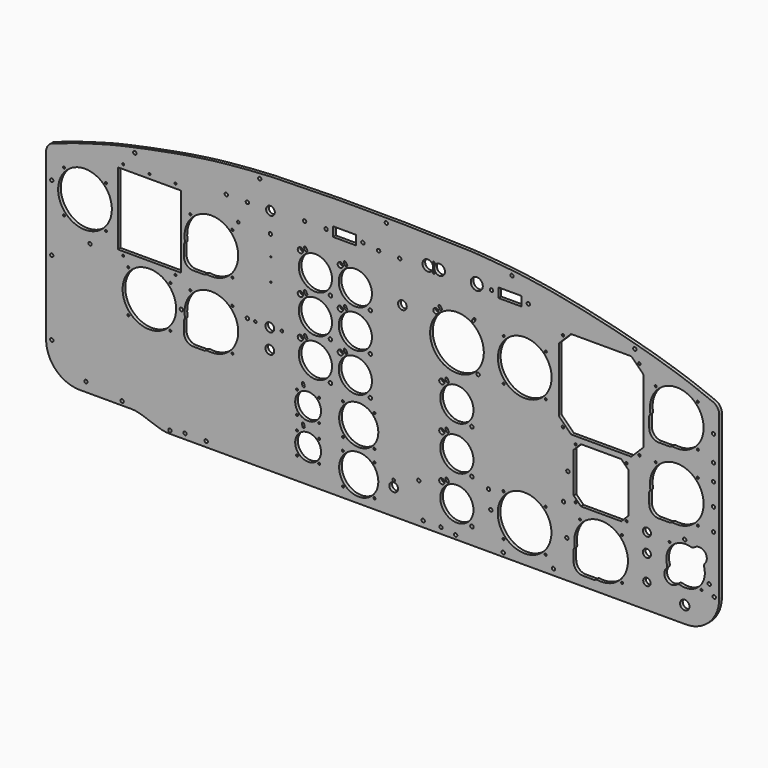
from build123d import *

# Parameters (mm, degrees)
F0_R     = 2.5
F0_R_2   = 1.5
F0_R_3   = 29.25
F0_R_4   = 19.3
F0_R_5   = 39.95
F0_R_6   = 2.6
F0_R_7   = 6.5
F0_R_8   = 2
F0_R_9   = 24.8
F0_R_10  = 3.95
F0_R_11  = 40.1
F0_R_12  = 5.5
F0_R_13  = 7
F0_R_14  = 6
F0_W     = 94
F0_H     = 108
F0_R_15  = 1
F0_W_2   = 34
F0_H_2   = 14
F0_R_16  = 1.8
F0_R_17  = 8
F0_R_18  = 9
F1_DEPTH = 5


# Not quite as in the source:
# - ends of sketch curves that miss each other by under 0.0002 mm in the source are joined
# - a feature names something its author has since deleted; it is built from what else it names


with BuildPart() as f1:
    # F0 (on Front) → F1 (new body)
    with BuildSketch(Plane.XZ):
        with BuildLine():
            ThreePointArc((135.741569039, 191.2079776505), (132.6141103531, 191.3792452145), (129.4850340278, 191.5178517119))
            ThreePointArc((129.4850340278, 191.5178517119), (-17.7264600255, 194.6267238973), (-164.9547639998, 192.4551859949))
            Line((-164.9547639998, 192.4551859949), (-191.066396, 190.888488))
            ThreePointArc((-191.066396, 190.888488), (-199.9950090203, 190.2859144937), (-208.9136419356, 189.5502432845))
            Line((-208.9136419356, 189.5502432845), (-232.326729, 187.443066))
            ThreePointArc((-232.326729, 187.443066), (-249.9687704393, 185.5919994012), (-267.5483811225, 183.2202148163))
            Line((-267.5483811225, 183.2202148163), (-288.605712, 180.061615))
            ThreePointArc((-288.605712, 180.061615), (-299.9814935886, 178.2434149523), (-311.3202700448, 176.2071422363))
            Line((-311.3202700448, 176.2071422363), (-344.055131, 170.003487))
            ThreePointArc((-344.055131, 170.003487), (-349.9940173558, 168.8469464334), (-355.9209391639, 167.6305767785))
            Line((-355.9209391639, 167.6305767785), (-380.749966, 162.404369))
            ThreePointArc((-380.749966, 162.404369), (-399.923291883, 158.0393315675), (-418.9432839055, 153.0483516623))
            Line((-418.9432839055, 153.0483516623), (-436.763326, 148.05874))
            ThreePointArc((-436.763326, 148.05874), (-449.9540896327, 144.201879695), (-463.0530571075, 140.0439153256))
            Line((-463.0530571075, 140.0439153256), (-492.340506, 130.376708))
            ThreePointArc((-492.340506, 130.376708), (-499.6985161403, 124.9082347034), (-502.5, 116.179191))
            Line((-502.5, 116.179191), (-502.5, -130.647528))
            ThreePointArc((-502.5, -130.647528), (-487.8553390593, -166.0028670593), (-452.5, -180.647528))
            Line((-452.5, -180.647528), (-375.801279, -180.647528))
            ThreePointArc((-375.801279, -180.647528), (-367.6120980534, -181.3227136017), (-359.6440857893, -183.3300353831))
            Line((-359.6440857893, -183.3300353831), (-334.355914, -191.965021))
            ThreePointArc((-334.355914, -191.965021), (-326.3879017872, -193.9723424247), (-318.198721, -194.647528))
            Line((-318.198721, -194.647528), (452.5, -194.647528))
            ThreePointArc((452.5, -194.647528), (487.8553390593, -180.0028670593), (502.5, -144.647528))
            Line((502.5, -144.647528), (502.5, 97.162105))
            ThreePointArc((502.5, 97.162105), (499.8924727989, 105.6135319758), (492.976450943, 111.1266488547))
            Line((492.976450943, 111.1266488547), (469.730257, 120.173737))
            ThreePointArc((469.730257, 120.173737), (449.8769209382, 127.4999158755), (429.7775799751, 134.1214219196))
            Line((429.7775799751, 134.1214219196), (410.573025, 140.074834))
            ThreePointArc((410.573025, 140.074834), (399.9715720426, 143.2544076566), (389.3132729084, 146.2378876609))
            Line((389.3132729084, 146.2378876609), (360.903911, 153.908416))
            ThreePointArc((360.903911, 153.908416), (349.9742295543, 156.7493500292), (338.9930159808, 159.3840779165))
            Line((338.9930159808, 159.3840779165), (308.383551, 166.424255))
            ThreePointArc((308.383551, 166.424255), (299.9870413401, 168.2921835026), (291.5646160829, 170.0395484146))
            Line((291.5646160829, 170.0395484146), (264.271898, 175.498092))
            ThreePointArc((264.271898, 175.498092), (249.9695922042, 178.1786072411), (235.6064889537, 180.5114976916))
            Line((235.6064889537, 180.5114976916), (217.548382, 183.220214))
            ThreePointArc((217.548382, 183.220214), (199.9687714246, 185.5919992831), (182.3267300249, 187.4430662765))
            Line((182.3267300249, 187.4430662765), (158.913642, 189.550244))
            ThreePointArc((158.913642, 189.550244), (149.9950095181, 190.2859144564), (141.0663969549, 190.8884872484))
            Line((141.0663969549, 190.8884872484), (135.741569039, 191.2079776505))
        make_face()
        with Locations((-389, -174.647528)):
            Circle(F0_R, mode=Mode.SUBTRACT)
        with Locations((-443, -166.647528)):
            Circle(F0_R, mode=Mode.SUBTRACT)
        with Locations((-317.5, -190.147528)):
            Circle(F0_R, mode=Mode.SUBTRACT)
        with Locations((-295, -186.647528)):
            Circle(F0_R, mode=Mode.SUBTRACT)
        with Locations((-263.5, -186.647528)):
            Circle(F0_R, mode=Mode.SUBTRACT)
        with Locations((-494, -128.647528)):
            Circle(F0_R, mode=Mode.SUBTRACT)
        with Locations((-127.881654, -161.579183)):
            Circle(F0_R_2, mode=Mode.SUBTRACT)
        with Locations((-59.3, -179.947528)):
            Circle(F0_R_2, mode=Mode.SUBTRACT)
        with Locations((-12.2, -179.947528)):
            Circle(F0_R_2, mode=Mode.SUBTRACT)
        with Locations((-94.718346, -161.579183)):
            Circle(F0_R_2, mode=Mode.SUBTRACT)
        with Locations((-35.75, -156.397528)):
            Circle(F0_R_3, mode=Mode.SUBTRACT)
        with Locations((-127.881654, -128.415874)):
            Circle(F0_R_2, mode=Mode.SUBTRACT)
        with Locations((-127.881654, -107.979183)):
            Circle(F0_R_2, mode=Mode.SUBTRACT)
        with Locations((-111.3, -144.997528)):
            Circle(F0_R_4, mode=Mode.SUBTRACT)
        with Locations((-94.718346, -128.415874)):
            Circle(F0_R_2, mode=Mode.SUBTRACT)
        with Locations((-59.3, -132.847528)):
            Circle(F0_R_2, mode=Mode.SUBTRACT)
        with Locations((-12.2, -132.847528)):
            Circle(F0_R_2, mode=Mode.SUBTRACT)
        with BuildLine():
            ThreePointArc((-116.3510682855, -119.9195418044), (-117.5768700198, -122.0695354275), (-119.7268511404, -120.8437117647))
            Line((-119.7268511404, -120.8437117647), (-120.650987, -117.467919))
            ThreePointArc((-120.650987, -117.467919), (-119.4175845384, -115.3159006328), (-117.2711185731, -116.5589411514))
            Line((-117.2711185731, -116.5589411514), (-116.3510682855, -119.9195418044))
        make_face(mode=Mode.SUBTRACT)
        with Locations((-94.718346, -107.979183)):
            Circle(F0_R_2, mode=Mode.SUBTRACT)
        with Locations((-59.3, -114.947528)):
            Circle(F0_R_2, mode=Mode.SUBTRACT)
        with Locations((-12.2, -114.947528)):
            Circle(F0_R_2, mode=Mode.SUBTRACT)
        with Locations((-379.730896, -58.878425)):
            Circle(F0_R_2, mode=Mode.SUBTRACT)
        with Locations((-316.869103, -58.878425)):
            Circle(F0_R_2, mode=Mode.SUBTRACT)
        with Locations((-494, -17.147528)):
            Circle(F0_R, mode=Mode.SUBTRACT)
        with Locations((-348.3, -27.447528)):
            Circle(F0_R_5, mode=Mode.SUBTRACT)
        with Locations((-300.5, -25.647528)):
            Circle(F0_R, mode=Mode.SUBTRACT)
        with BuildLine():
            ThreePointArc((-264.6933823946, -68.0597605441), (-265.3038534949, -68.4216231267), (-266.002257, -68.547528))
            Line((-266.002257, -68.547528), (-282.6, -68.547528))
            ThreePointArc((-282.6, -68.547528), (-292.6409162928, -64.3884442928), (-296.8, -54.347528))
            Line((-296.8, -54.347528), (-296.8, -38.547528))
            ThreePointArc((-296.8, -38.547528), (-296.6647556198, -37.8245574071), (-296.2773135218, -37.1993645239))
            ThreePointArc((-296.2773135218, -37.1993645239), (-295.3984169479, -35.6450094204), (-295.2834646323, -33.8630821025))
            ThreePointArc((-295.2834646323, -33.8630821025), (-227.5670304906, 1.1277414928), (-261.4973429879, -67.1262479174))
            ThreePointArc((-261.4973429879, -67.1262479174), (-263.1971096036, -67.2446562762), (-264.6933823946, -68.0597605441))
        make_face(mode=Mode.SUBTRACT)
        with Locations((-127.881654, -74.815874)):
            Circle(F0_R_2, mode=Mode.SUBTRACT)
        with Locations((-224.269103, -58.878425)):
            Circle(F0_R_2, mode=Mode.SUBTRACT)
        with Locations((-111.3, -91.397528)):
            Circle(F0_R_4, mode=Mode.SUBTRACT)
        with Locations((-94.718346, -74.815874)):
            Circle(F0_R_2, mode=Mode.SUBTRACT)
        with Locations((-35.75, -91.397528)):
            Circle(F0_R_3, mode=Mode.SUBTRACT)
        with BuildLine():
            ThreePointArc((-116.3510682855, -66.3195418044), (-117.5768700198, -68.4695354275), (-119.7268511404, -67.2437117647))
            Line((-119.7268511404, -67.2437117647), (-120.650987, -63.867919))
            ThreePointArc((-120.650987, -63.867919), (-119.4175845384, -61.7159006328), (-117.2711185731, -62.9589411514))
            Line((-117.2711185731, -62.9589411514), (-116.3510682855, -66.3195418044))
        make_face(mode=Mode.SUBTRACT)
        with Locations((-77.949362, -49.898169)):
            Circle(F0_R_6, mode=Mode.SUBTRACT)
        with Locations((-59.3, -67.847528)):
            Circle(F0_R_2, mode=Mode.SUBTRACT)
        with Locations((-12.2, -67.847528)):
            Circle(F0_R_2, mode=Mode.SUBTRACT)
        with Locations((-18.349362, -49.898169)):
            Circle(F0_R_6, mode=Mode.SUBTRACT)
        with Locations((-168.5, -35.647528)):
            Circle(F0_R_7, mode=Mode.SUBTRACT)
        with Locations((-202, -5.147528)):
            Circle(F0_R, mode=Mode.SUBTRACT)
        with Locations((-190, -5.647528)):
            Circle(F0_R_8, mode=Mode.SUBTRACT)
        with Locations((-168.5, -6.147528)):
            Circle(F0_R_7, mode=Mode.SUBTRACT)
        with Locations((-150.5, -5.147528)):
            Circle(F0_R_8, mode=Mode.SUBTRACT)
        with Locations((-100.400003, -27.447528)):
            Circle(F0_R_9, mode=Mode.SUBTRACT)
        with Locations((-40.800003, -27.447528)):
            Circle(F0_R_9, mode=Mode.SUBTRACT)
        with Locations((-122.850643, -4.996888)):
            Circle(F0_R_10, mode=Mode.SUBTRACT)
        with BuildLine():
            ThreePointArc((-112.6555519379, -1.6024819658), (-113.3428170619, -3.9800283878), (-115.7203567133, -3.2927398419))
            Line((-115.7203567133, -3.2927398419), (-117.410584, -0.227918))
            ThreePointArc((-117.410584, -0.227918), (-116.7164059044, 2.1533814048), (-114.3382438007, 1.4485311076))
            Line((-114.3382438007, 1.4485311076), (-112.6555519379, -1.6024819658))
        make_face(mode=Mode.SUBTRACT)
        with Locations((-63.250643, -4.996888)):
            Circle(F0_R_10, mode=Mode.SUBTRACT)
        with BuildLine():
            ThreePointArc((-53.0555519379, -1.6024819658), (-53.7428170619, -3.9800283878), (-56.1203567133, -3.2927398419))
            Line((-56.1203567133, -3.2927398419), (-57.810584, -0.227918))
            ThreePointArc((-57.810584, -0.227918), (-57.1164059044, 2.1533814048), (-54.7382438007, 1.4485311076))
            Line((-54.7382438007, 1.4485311076), (-53.0555519379, -1.6024819658))
        make_face(mode=Mode.SUBTRACT)
        with Locations((60.5, -185.647528)):
            Circle(F0_R, mode=Mode.SUBTRACT)
        with Locations((87, -185.647528)):
            Circle(F0_R, mode=Mode.SUBTRACT)
        with Locations((109, -188.647528)):
            Circle(F0_R, mode=Mode.SUBTRACT)
        with Locations((16.5, -156.147528)):
            Circle(F0_R_7, mode=Mode.SUBTRACT)
        with Locations((16.5, -146.647528)):
            Circle(F0_R_8, mode=Mode.SUBTRACT)
        with Locations((110.8, -147.347528)):
            Circle(F0_R_9, mode=Mode.SUBTRACT)
        with Locations((180, -188.647528)):
            Circle(F0_R, mode=Mode.SUBTRACT)
        with Locations((180.419104, -170.978425)):
            Circle(F0_R_2, mode=Mode.SUBTRACT)
        with Locations((243.280897, -170.978425)):
            Circle(F0_R_2, mode=Mode.SUBTRACT)
        with Locations((133.250641, -169.798169)):
            Circle(F0_R_6, mode=Mode.SUBTRACT)
        with Locations((54, -135.147528)):
            Circle(F0_R, mode=Mode.SUBTRACT)
        with Locations((88.34936, -124.896888)):
            Circle(F0_R_10, mode=Mode.SUBTRACT)
        with BuildLine():
            ThreePointArc((98.5444510621, -121.5024819658), (97.8571859381, -123.8800283878), (95.4796462867, -123.1927398419))
            Line((95.4796462867, -123.1927398419), (93.789419, -120.127918))
            ThreePointArc((93.789419, -120.127918), (94.4835970956, -117.7466185952), (96.8617591993, -118.4514688924))
            Line((96.8617591993, -118.4514688924), (98.5444510621, -121.5024819658))
        make_face(mode=Mode.SUBTRACT)
        with Locations((161.5, -138.647528)):
            Circle(F0_R, mode=Mode.SUBTRACT)
        with Locations((211.85, -139.547528)):
            Circle(F0_R_11, mode=Mode.SUBTRACT)
        with Locations((158, -112.647528)):
            Circle(F0_R, mode=Mode.SUBTRACT)
        with Locations((133.250641, -104.198169)):
            Circle(F0_R_6, mode=Mode.SUBTRACT)
        with Locations((180.419104, -108.116632)):
            Circle(F0_R_2, mode=Mode.SUBTRACT)
        with Locations((243.280897, -108.116632)):
            Circle(F0_R_2, mode=Mode.SUBTRACT)
        with Locations((255, -185.647528)):
            Circle(F0_R, mode=Mode.SUBTRACT)
        with Locations((357.530897, -170.978425)):
            Circle(F0_R_2, mode=Mode.SUBTRACT)
        with Locations((394.5, -157.647528)):
            Circle(F0_R_12, mode=Mode.SUBTRACT)
        with Locations((451, -169.647528)):
            Circle(F0_R_13, mode=Mode.SUBTRACT)
        with Locations((275, -138.647528)):
            Circle(F0_R, mode=Mode.SUBTRACT)
        with BuildLine():
            ThreePointArc((317.1066176054, -180.1597605441), (316.4961465051, -180.5216231267), (315.797743, -180.647528))
            Line((315.797743, -180.647528), (299.2, -180.647528))
            ThreePointArc((299.2, -180.647528), (289.1590837072, -176.4884442928), (285, -166.447528))
            Line((285, -166.447528), (285, -150.647528))
            ThreePointArc((285, -150.647528), (285.1352443802, -149.9245574071), (285.5226864782, -149.2993645239))
            ThreePointArc((285.5226864782, -149.2993645239), (286.4015830521, -147.7450094204), (286.5165353677, -145.9630821025))
            ThreePointArc((286.5165353677, -145.9630821025), (354.2329695094, -110.9722585072), (320.3026570121, -179.2262479174))
            ThreePointArc((320.3026570121, -179.2262479174), (318.6028903964, -179.3446562762), (317.1066176054, -180.1597605441))
        make_face(mode=Mode.SUBTRACT)
        with Locations((294.669104, -108.116632)):
            Circle(F0_R_2, mode=Mode.SUBTRACT)
        with Locations((357.530897, -108.116632)):
            Circle(F0_R_2, mode=Mode.SUBTRACT)
        with Locations((476, -141.647528)):
            Circle(F0_R_2, mode=Mode.SUBTRACT)
        with Locations((495, -144.647528)):
            Circle(F0_R, mode=Mode.SUBTRACT)
        with Locations((487.5, -130.147528)):
            Circle(F0_R, mode=Mode.SUBTRACT)
        with Locations((394.5, -120.147528)):
            Circle(F0_R_14, mode=Mode.SUBTRACT)
        with BuildLine():
            ThreePointArc((479.9020604453, -110.0282171579), (472.4459566685, -138.3593420507), (444.0197490276, -145.4443149076))
            ThreePointArc((444.0197490276, -145.4443149076), (441.5053900455, -145.3537612476), (439.2652582695, -146.499191303))
            ThreePointArc((439.2652582695, -146.499191303), (423.7813893308, -145.9962507879), (423.4809780694, -130.5071290634))
            ThreePointArc((423.4809780694, -130.5071290634), (424.6556053692, -128.2821680605), (424.5979402014, -125.7668399427))
            ThreePointArc((424.5979402014, -125.7668399427), (432.0540429937, -97.4357142827), (460.4802512467, -90.3507411744))
            ThreePointArc((460.4802512467, -90.3507411744), (462.9946104868, -90.4412958561), (465.2347427305, -89.295865697))
            ThreePointArc((465.2347427305, -89.295865697), (480.7186109317, -89.798806478), (481.0190219306, -105.2879279366))
            ThreePointArc((481.0190219306, -105.2879279366), (479.8443955535, -107.5128892677), (479.9020604453, -110.0282171579))
        make_face(mode=Mode.SUBTRACT)
        with Locations((110.8, -81.747528)):
            Circle(F0_R_9, mode=Mode.SUBTRACT)
        with Locations((88.34936, -59.296888)):
            Circle(F0_R_10, mode=Mode.SUBTRACT)
        with BuildLine():
            ThreePointArc((98.5444510621, -55.9024819658), (97.8571859381, -58.2800283878), (95.4796462867, -57.5927398419))
            Line((95.4796462867, -57.5927398419), (93.789419, -54.527918))
            ThreePointArc((93.789419, -54.527918), (94.4835970956, -52.1466185952), (96.8617591993, -52.8514688924))
            Line((96.8617591993, -52.8514688924), (98.5444510621, -55.9024819658))
        make_face(mode=Mode.SUBTRACT)
        with Locations((110.8, -16.147528)):
            Circle(F0_R_9, mode=Mode.SUBTRACT)
        with Locations((133.250641, -38.598169)):
            Circle(F0_R_6, mode=Mode.SUBTRACT)
        with Locations((270, -92.647528)):
            Circle(F0_R, mode=Mode.SUBTRACT)
        with Locations((287.995773, -87.63635)):
            Circle(F0_R_2, mode=Mode.SUBTRACT)
        with Locations((364.198177, -87.63635)):
            Circle(F0_R_2, mode=Mode.SUBTRACT)
        with Locations((276.5, -50.647528)):
            Circle(F0_R, mode=Mode.SUBTRACT)
        Polygon((285.199997, -19.462587), (295.999987, -8.648008), (356.186954, -8.648008), (367.000807, -19.447999), (366.999997, -79.63586), (356.200003, -90.447049), (295.999997, -90.448008), (285.199997, -79.648008), align=None, mode=Mode.SUBTRACT)
        with Locations((394.5, -92.147528)):
            Circle(F0_R_14, mode=Mode.SUBTRACT)
        with Locations((428.5, -94.147528)):
            Circle(F0_R_2, mode=Mode.SUBTRACT)
        with Locations((451, -83.647528)):
            Circle(F0_R, mode=Mode.SUBTRACT)
        with Locations((470.530897, -58.878425)):
            Circle(F0_R_2, mode=Mode.SUBTRACT)
        with Locations((494, -59.647528)):
            Circle(F0_R, mode=Mode.SUBTRACT)
        with Locations((287.995773, -11.43635)):
            Circle(F0_R_2, mode=Mode.SUBTRACT)
        with Locations((364.195773, -11.43635)):
            Circle(F0_R_2, mode=Mode.SUBTRACT)
        with BuildLine():
            ThreePointArc((430.1066176054, -68.0597605441), (429.4961465051, -68.4216231267), (428.797743, -68.547528))
            Line((428.797743, -68.547528), (412.2, -68.547528))
            ThreePointArc((412.2, -68.547528), (402.1590837072, -64.3884442928), (398, -54.347528))
            Line((398, -54.347528), (398, -38.547528))
            ThreePointArc((398, -38.547528), (398.1352443802, -37.8245574071), (398.5226864782, -37.1993645239))
            ThreePointArc((398.5226864782, -37.1993645239), (399.4015830521, -35.6450094204), (399.5165353677, -33.8630821025))
            ThreePointArc((399.5165353677, -33.8630821025), (467.2329695094, 1.1277414928), (433.3026570121, -67.1262479174))
            ThreePointArc((433.3026570121, -67.1262479174), (431.6028903964, -67.2446562762), (430.1066176054, -68.0597605441))
        make_face(mode=Mode.SUBTRACT)
        with Locations((494, -26.647528)):
            Circle(F0_R, mode=Mode.SUBTRACT)
        with Locations((-379.730896, 3.983368)):
            Circle(F0_R_2, mode=Mode.SUBTRACT)
        with Locations((-437, 16.352472)):
            Circle(F0_R, mode=Mode.SUBTRACT)
        with Locations((-387.3, 17.002472)):
            Circle(F0_R_2, mode=Mode.SUBTRACT)
        with Locations((-475.830896, 41.021575)):
            Circle(F0_R_2, mode=Mode.SUBTRACT)
        with Locations((-412.969103, 41.021575)):
            Circle(F0_R_2, mode=Mode.SUBTRACT)
        with Locations((-316.869103, 3.983368)):
            Circle(F0_R_2, mode=Mode.SUBTRACT)
        with Locations((-287.130896, 3.983368)):
            Circle(F0_R_2, mode=Mode.SUBTRACT)
        with Locations((-309.3, 17.002472)):
            Circle(F0_R_2, mode=Mode.SUBTRACT)
        with Locations((-444.4, 72.452472)):
            Circle(F0_R_11, mode=Mode.SUBTRACT)
        with Locations((-494, 81.352472)):
            Circle(F0_R, mode=Mode.SUBTRACT)
        with BuildLine():
            ThreePointArc((-264.6933823946, 31.8402394559), (-265.3038534949, 31.4783768733), (-266.002257, 31.352472))
            Line((-266.002257, 31.352472), (-282.6, 31.352472))
            ThreePointArc((-282.6, 31.352472), (-292.6409162928, 35.5115557072), (-296.8, 45.552472))
            Line((-296.8, 45.552472), (-296.8, 61.352472))
            ThreePointArc((-296.8, 61.352472), (-296.6647556198, 62.0754425929), (-296.2773135218, 62.7006354761))
            ThreePointArc((-296.2773135218, 62.7006354761), (-295.3984169479, 64.2549905796), (-295.2834646323, 66.0369178975))
            ThreePointArc((-295.2834646323, 66.0369178975), (-227.5670304906, 101.0277414928), (-261.4973429879, 32.7737520826))
            ThreePointArc((-261.4973429879, 32.7737520826), (-263.1971096036, 32.6553437238), (-264.6933823946, 31.8402394559))
        make_face(mode=Mode.SUBTRACT)
        with Locations((-348.3, 76.502472)):
            Rectangle(F0_W, F0_H, mode=Mode.SUBTRACT)
        with Locations((-224.269103, 3.983368)):
            Circle(F0_R_2, mode=Mode.SUBTRACT)
        with Locations((-224.269103, 41.021575)):
            Circle(F0_R_2, mode=Mode.SUBTRACT)
        with Locations((-77.949359, 7.601831)):
            Circle(F0_R_6, mode=Mode.SUBTRACT)
        with Locations((-18.349359, 7.601831)):
            Circle(F0_R_6, mode=Mode.SUBTRACT)
        with Locations((-100.4, 30.052472)):
            Circle(F0_R_9, mode=Mode.SUBTRACT)
        with Locations((-40.8, 30.052472)):
            Circle(F0_R_9, mode=Mode.SUBTRACT)
        with Locations((-167, 53.852472)):
            Circle(F0_R_15, mode=Mode.SUBTRACT)
        with Locations((-167, 86.852472)):
            Circle(F0_R_15, mode=Mode.SUBTRACT)
        with Locations((-122.85064, 52.503112)):
            Circle(F0_R_10, mode=Mode.SUBTRACT)
        with BuildLine():
            ThreePointArc((-112.6555489379, 55.8975180342), (-113.3428140619, 53.5199716122), (-115.7203537133, 54.2072601581))
            Line((-115.7203537133, 54.2072601581), (-117.410581, 57.272082))
            ThreePointArc((-117.410581, 57.272082), (-116.7164029044, 59.6533814048), (-114.3382408007, 58.9485311076))
            Line((-114.3382408007, 58.9485311076), (-112.6555489379, 55.8975180342))
        make_face(mode=Mode.SUBTRACT)
        with Locations((-63.25064, 52.503112)):
            Circle(F0_R_10, mode=Mode.SUBTRACT)
        with Locations((-77.949359, 65.101831)):
            Circle(F0_R_6, mode=Mode.SUBTRACT)
        with BuildLine():
            ThreePointArc((-53.0555489379, 55.8975180342), (-53.7428140619, 53.5199716122), (-56.1203537133, 54.2072601581))
            Line((-56.1203537133, 54.2072601581), (-57.810581, 57.272082))
            ThreePointArc((-57.810581, 57.272082), (-57.1164029044, 59.6533814048), (-54.7382408007, 58.9485311076))
            Line((-54.7382408007, 58.9485311076), (-53.0555489379, 55.8975180342))
        make_face(mode=Mode.SUBTRACT)
        with Locations((-18.349359, 65.101831)):
            Circle(F0_R_6, mode=Mode.SUBTRACT)
        with Locations((-100.4, 87.552472)):
            Circle(F0_R_9, mode=Mode.SUBTRACT)
        with Locations((-40.8, 87.552472)):
            Circle(F0_R_9, mode=Mode.SUBTRACT)
        with Locations((-475.830896, 103.883368)):
            Circle(F0_R_2, mode=Mode.SUBTRACT)
        with Locations((-412.969103, 103.883368)):
            Circle(F0_R_2, mode=Mode.SUBTRACT)
        with Locations((-387.3, 137.002472)):
            Circle(F0_R_2, mode=Mode.SUBTRACT)
        with Locations((-287.130896, 103.883368)):
            Circle(F0_R_2, mode=Mode.SUBTRACT)
        with Locations((-348.3, 137.002472)):
            Circle(F0_R_2, mode=Mode.SUBTRACT)
        with Locations((-309.3, 137.002472)):
            Circle(F0_R_2, mode=Mode.SUBTRACT)
        with Locations((-370, 157.667106)):
            Circle(F0_R, mode=Mode.SUBTRACT)
        with Locations((-224.269103, 103.883368)):
            Circle(F0_R_2, mode=Mode.SUBTRACT)
        with Locations((-215.5, 116.852472)):
            Circle(F0_R_8, mode=Mode.SUBTRACT)
        with Locations((-167.5, 116.852472)):
            Circle(F0_R, mode=Mode.SUBTRACT)
        with Locations((-122.85064, 110.003112)):
            Circle(F0_R_10, mode=Mode.SUBTRACT)
        with BuildLine():
            ThreePointArc((-112.6555489379, 113.3975180342), (-113.3428140619, 111.0199716122), (-115.7203537133, 111.7072601581))
            Line((-115.7203537133, 111.7072601581), (-117.410581, 114.772082))
            ThreePointArc((-117.410581, 114.772082), (-116.7164029044, 117.1533814048), (-114.3382408007, 116.4485311076))
            Line((-114.3382408007, 116.4485311076), (-112.6555489379, 113.3975180342))
        make_face(mode=Mode.SUBTRACT)
        with Locations((-63.25064, 110.003112)):
            Circle(F0_R_10, mode=Mode.SUBTRACT)
        with BuildLine():
            ThreePointArc((-53.0555489379, 113.3975180342), (-53.7428140619, 111.0199716122), (-56.1203537133, 111.7072601581))
            Line((-56.1203537133, 111.7072601581), (-57.810581, 114.772082))
            ThreePointArc((-57.810581, 114.772082), (-57.1164029044, 117.1533814048), (-54.7382408007, 116.4485311076))
            Line((-54.7382408007, 116.4485311076), (-53.0555489379, 113.3975180342))
        make_face(mode=Mode.SUBTRACT)
        with Locations((-233.5, 147.352472)):
            Circle(F0_R, mode=Mode.SUBTRACT)
        with Locations((-202, 147.352472)):
            Circle(F0_R, mode=Mode.SUBTRACT)
        with Locations((-167.5, 147.352472)):
            Circle(F0_R_7, mode=Mode.SUBTRACT)
        with Locations((-183.5, 184.342472)):
            Circle(F0_R, mode=Mode.SUBTRACT)
        with Locations((-116.5, 150.352472)):
            Circle(F0_R, mode=Mode.SUBTRACT)
        with Locations((-84.5, 150.352472)):
            Circle(F0_R, mode=Mode.SUBTRACT)
        with Locations((-57, 150.352472)):
            Rectangle(F0_W_2, F0_H_2, mode=Mode.SUBTRACT)
        with Locations((-29.5, 150.352472)):
            Circle(F0_R, mode=Mode.SUBTRACT)
        with Locations((-6, 147.352472)):
            Circle(F0_R, mode=Mode.SUBTRACT)
        with Locations((88.34936, 6.303112)):
            Circle(F0_R_10, mode=Mode.SUBTRACT)
        with BuildLine():
            ThreePointArc((98.5444510621, 9.6975180342), (97.8571859381, 7.3199716122), (95.4796462867, 8.0072601581))
            Line((95.4796462867, 8.0072601581), (93.789419, 11.072082))
            ThreePointArc((93.789419, 11.072082), (94.4835970956, 13.4533814048), (96.8617591993, 12.7485311076))
            Line((96.8617591993, 12.7485311076), (98.5444510621, 9.6975180342))
        make_face(mode=Mode.SUBTRACT)
        with Locations((142.380897, 33.171575)):
            Circle(F0_R_6, mode=Mode.SUBTRACT)
        with Locations((180.719104, 33.171575)):
            Circle(F0_R_2, mode=Mode.SUBTRACT)
        with Locations((243.580897, 33.171575)):
            Circle(F0_R_2, mode=Mode.SUBTRACT)
        with Locations((110.95, 64.602472)):
            Circle(F0_R_11, mode=Mode.SUBTRACT)
        with Locations((29.5, 87.352472)):
            Circle(F0_R_7, mode=Mode.SUBTRACT)
        with Locations((79.519104, 96.033368)):
            Circle(F0_R_10, mode=Mode.SUBTRACT)
        with Locations((212.15, 64.602472)):
            Circle(F0_R_11, mode=Mode.SUBTRACT)
        with Locations((180.719104, 96.033368)):
            Circle(F0_R_2, mode=Mode.SUBTRACT)
        with Locations((243.580897, 96.033368)):
            Circle(F0_R_2, mode=Mode.SUBTRACT)
        with Locations((269.15, 5.052472)):
            Circle(F0_R_16, mode=Mode.SUBTRACT)
        with Locations((383.35, 5.052472)):
            Circle(F0_R_16, mode=Mode.SUBTRACT)
        with Locations((407.669104, 3.983368)):
            Circle(F0_R_2, mode=Mode.SUBTRACT)
        with Locations((470.530897, 3.983368)):
            Circle(F0_R_2, mode=Mode.SUBTRACT)
        with Locations((494, 6.352472)):
            Circle(F0_R, mode=Mode.SUBTRACT)
        with Locations((494, 31.352472)):
            Circle(F0_R, mode=Mode.SUBTRACT)
        with Locations((470.530897, 41.021575)):
            Circle(F0_R_2, mode=Mode.SUBTRACT)
        with BuildLine():
            Line((280.664214, -0.061742), (263.835787, 16.766685))
            ThreePointArc((263.835787, 16.766685), (263.4022410703, 17.4155318086), (263.25, 18.180899))
            Line((263.25, 18.180899), (263.25, 112.524044))
            ThreePointArc((263.25, 112.524044), (263.4022410703, 113.2894111914), (263.8357869376, 113.9382580624))
            Line((263.8357869376, 113.9382580624), (280.664214, 130.766685))
            ThreePointArc((280.664214, 130.766685), (281.3130601353, 131.200231065), (282.078427, 131.352472))
            Line((282.078427, 131.352472), (370.421573, 131.352472))
            ThreePointArc((370.421573, 131.352472), (371.1869401914, 131.2002309297), (371.8357870624, 130.7666850624))
            Line((371.8357870624, 130.7666850624), (388.664214, 113.938258))
            ThreePointArc((388.664214, 113.938258), (389.097759065, 113.2894108647), (389.25, 112.524044))
            Line((389.25, 112.524044), (389.25, 18.180899))
            ThreePointArc((389.25, 18.180899), (389.097759065, 17.4155321353), (388.6642135624, 16.7666854376))
            Line((388.6642135624, 16.7666854376), (371.835787, -0.061742))
            ThreePointArc((371.835787, -0.061742), (371.1869398647, -0.495287065), (370.421573, -0.647528))
            Line((370.421573, -0.647528), (282.078427, -0.647528))
            ThreePointArc((282.078427, -0.647528), (281.3130604619, -0.4952872003), (280.664214, -0.061742))
        make_face(mode=Mode.SUBTRACT)
        with BuildLine():
            ThreePointArc((430.1066176054, 31.8402394559), (429.4961465051, 31.4783768733), (428.797743, 31.352472))
            Line((428.797743, 31.352472), (412.2, 31.352472))
            ThreePointArc((412.2, 31.352472), (402.1590837072, 35.5115557072), (398, 45.552472))
            Line((398, 45.552472), (398, 61.352472))
            ThreePointArc((398, 61.352472), (398.1352443802, 62.0754425929), (398.5226864782, 62.7006354761))
            ThreePointArc((398.5226864782, 62.7006354761), (399.4015830521, 64.2549905796), (399.5165353677, 66.0369178975))
            ThreePointArc((399.5165353677, 66.0369178975), (467.2329695094, 101.0277414928), (433.3026570121, 32.7737520826))
            ThreePointArc((433.3026570121, 32.7737520826), (431.6028903964, 32.6553437238), (430.1066176054, 31.8402394559))
        make_face(mode=Mode.SUBTRACT)
        with Locations((494, 69.352472)):
            Circle(F0_R, mode=Mode.SUBTRACT)
        with BuildLine():
            ThreePointArc((88.2096198934, 101.9578599292), (87.7196724878, 99.5319555183), (85.2937729302, 100.0219269537))
            Line((85.2937729302, 100.0219269537), (83.357869, 102.937793))
            ThreePointArc((83.357869, 102.937793), (83.8543978248, 105.368004215), (86.2823579527, 104.8605819692))
            Line((86.2823579527, 104.8605819692), (88.2096198934, 101.9578599292))
        make_face(mode=Mode.SUBTRACT)
        with Locations((76.25, 145.352472)):
            Circle(F0_R_2, mode=Mode.SUBTRACT)
        with BuildLine():
            Line((138.542131, 102.937793), (136.606227, 100.021927))
            ThreePointArc((136.606227, 100.021927), (134.1803272818, 99.5319556713), (133.6903804125, 101.95786039))
            Line((133.6903804125, 101.95786039), (135.617642, 104.860582))
            ThreePointArc((135.617642, 104.860582), (138.0456021752, 105.368004215), (138.542131, 102.937793))
        make_face(mode=Mode.SUBTRACT)
        with Locations((25.5, 147.352472)):
            Circle(F0_R, mode=Mode.SUBTRACT)
        with Locations((67.5, 151.852472)):
            Circle(F0_R_17, mode=Mode.SUBTRACT)
        with Locations((85, 151.852472)):
            Circle(F0_R_17, mode=Mode.SUBTRACT)
        with Locations((76.25, 158.352472)):
            Circle(F0_R_2, mode=Mode.SUBTRACT)
        with Locations((5.5, 187.487086)):
            Circle(F0_R, mode=Mode.SUBTRACT)
        with Locations((140.5, 151.352472)):
            Circle(F0_R_18, mode=Mode.SUBTRACT)
        with Locations((162.5, 150.352472)):
            Circle(F0_R, mode=Mode.SUBTRACT)
        with Locations((190, 150.352472)):
            Rectangle(F0_W_2, F0_H_2, mode=Mode.SUBTRACT)
        with Locations((217.5, 150.352472)):
            Circle(F0_R, mode=Mode.SUBTRACT)
        with Locations((193, 179.386221)):
            Circle(F0_R, mode=Mode.SUBTRACT)
        with Locations((269.15, 125.652472)):
            Circle(F0_R_16, mode=Mode.SUBTRACT)
        with Locations((376.5, 142.684442)):
            Circle(F0_R, mode=Mode.SUBTRACT)
        with Locations((407.669104, 103.883368)):
            Circle(F0_R_2, mode=Mode.SUBTRACT)
        with Locations((470.530897, 103.883368)):
            Circle(F0_R_2, mode=Mode.SUBTRACT)
        with Locations((383.35, 125.652472)):
            Circle(F0_R_16, mode=Mode.SUBTRACT)
    extrude(amount=-F1_DEPTH)


solid = f1.part
